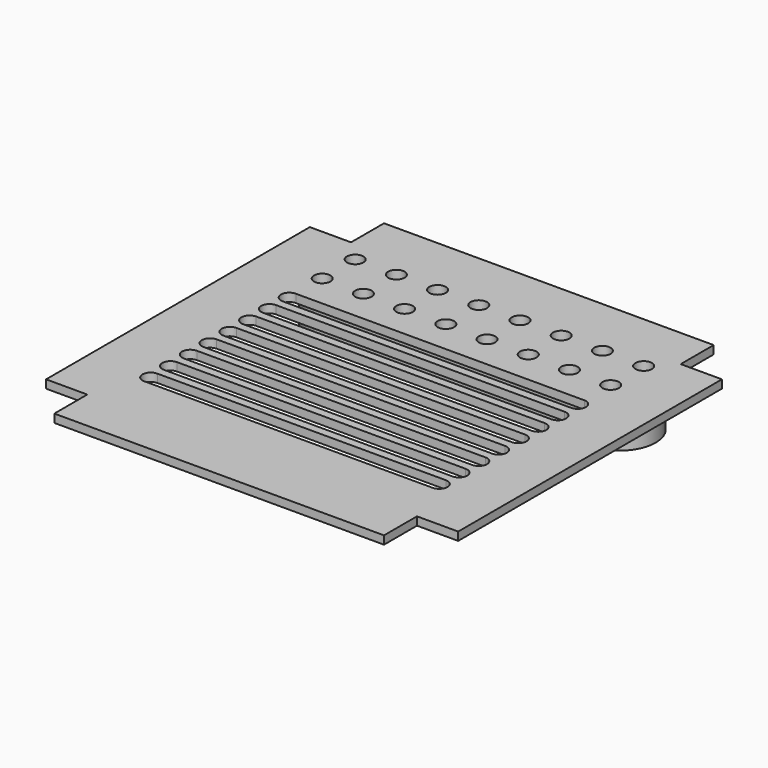
from build123d import *

# Parameters (mm, degrees)
F1_DEPTH = 2.54
F3_DEPTH = 12.7
F4_R     = 2.54
F5_DEPTH = 25.4


# Not quite as in the source:
# - a feature names something its author has since deleted; it is built from what else it names


with BuildPart() as f1:
    # F0 (on Top) → F1 (new body)
    with BuildSketch(Plane.XY):
        Polygon((50.8, 63.5), (0, 63.5), (-50.8, 63.5), (-50.8, 50.8), (-63.5, 50.8), (-63.5, 0), (-63.5, -50.8), (-50.8, -50.8), (-50.8, -63.5), (0, -63.5), (50.8, -63.5), (50.8, -50.8), (63.5, -50.8), (63.5, 0), (63.5, 50.8), (50.8, 50.8), align=None)
    extrude(amount=F1_DEPTH)

    # F2 (on face) → F3 (join)
    with BuildSketch(Plane(origin=(0, 0, 0), x_dir=(1, 0, 0), z_dir=(0, 0, -1))):
        with BuildLine():
            Line((43.2105347984, -26.8235280358), (-43.2105347984, -26.8235280358))
            ThreePointArc((-43.2105347984, -26.8235280358), (-53.3766044151, -38.3837321185), (-42.2611118031, -49.0342304111))
            Line((-42.2611118031, -49.0342304111), (42.2611118031, -49.0342304111))
            ThreePointArc((42.2611118031, -49.0342304111), (53.3766044151, -38.3837321185), (43.2105347984, -26.8235280358))
        make_face()
    extrude(amount=F3_DEPTH)

    # F4 (on face) → F5 (cut)
    with BuildSketch(Plane.XY.offset(2.54)):
        with Locations((-44.45, 44.45)):
            Circle(F4_R)
        with Locations((-44.45, 31.75)):
            Circle(F4_R)
        with Locations((-31.75, 44.45)):
            Circle(F4_R)
        with Locations((-31.75, 31.75)):
            Circle(F4_R)
        with Locations((-19.05, 44.45)):
            Circle(F4_R)
        with Locations((-19.05, 31.75)):
            Circle(F4_R)
        with Locations((-6.35, 44.45)):
            Circle(F4_R)
        with Locations((-6.35, 31.75)):
            Circle(F4_R)
        with Locations((6.35, 44.45)):
            Circle(F4_R)
        with Locations((6.35, 31.75)):
            Circle(F4_R)
        with Locations((19.05, 44.45)):
            Circle(F4_R)
        with Locations((19.05, 31.75)):
            Circle(F4_R)
        with Locations((31.75, 44.45)):
            Circle(F4_R)
        with Locations((31.75, 31.75)):
            Circle(F4_R)
        with Locations((44.45, 44.45)):
            Circle(F4_R)
        with Locations((44.45, 31.75)):
            Circle(F4_R)
        with BuildLine():
            Line((44.45, 21.59), (-44.45, 21.59))
            ThreePointArc((-44.45, 21.59), (-46.99, 19.05), (-44.45, 16.51))
            Line((-44.45, 16.51), (44.45, 16.51))
            ThreePointArc((44.45, 16.51), (46.99, 19.05), (44.45, 21.59))
        make_face()
        with BuildLine():
            Line((44.45, 13.97), (-44.45, 13.97))
            ThreePointArc((-44.45, 13.97), (-46.99, 11.43), (-44.45, 8.89))
            Line((-44.45, 8.89), (44.45, 8.89))
            ThreePointArc((44.45, 8.89), (46.99, 11.43), (44.45, 13.97))
        make_face()
        with BuildLine():
            Line((44.45, 6.35), (-44.45, 6.35))
            ThreePointArc((-44.45, 6.35), (-46.99, 3.81), (-44.45, 1.27))
            Line((-44.45, 1.27), (44.45, 1.27))
            ThreePointArc((44.45, 1.27), (46.99, 3.81), (44.45, 6.35))
        make_face()
        with BuildLine():
            Line((44.45, -1.27), (-44.45, -1.27))
            ThreePointArc((-44.45, -1.27), (-46.99, -3.81), (-44.45, -6.35))
            Line((-44.45, -6.35), (44.45, -6.35))
            ThreePointArc((44.45, -6.35), (46.99, -3.81), (44.45, -1.27))
        make_face()
        with BuildLine():
            Line((44.45, -8.89), (-44.45, -8.89))
            ThreePointArc((-44.45, -8.89), (-46.99, -11.43), (-44.45, -13.97))
            Line((-44.45, -13.97), (44.45, -13.97))
            ThreePointArc((44.45, -13.97), (46.99, -11.43), (44.45, -8.89))
        make_face()
        with BuildLine():
            Line((44.45, -16.51), (-44.45, -16.51))
            ThreePointArc((-44.45, -16.51), (-46.99, -19.05), (-44.45, -21.59))
            Line((-44.45, -21.59), (44.45, -21.59))
            ThreePointArc((44.45, -21.59), (46.99, -19.05), (44.45, -16.51))
        make_face()
        with BuildLine():
            Line((44.45, -24.13), (-44.45, -24.13))
            ThreePointArc((-44.45, -24.13), (-46.99, -26.67), (-44.45, -29.21))
            Line((-44.45, -29.21), (44.45, -29.21))
            ThreePointArc((44.45, -29.21), (46.99, -26.67), (44.45, -24.13))
        make_face()
        with BuildLine():
            Line((44.45, -31.75), (-44.45, -31.75))
            ThreePointArc((-44.45, -31.75), (-46.99, -34.29), (-44.45, -36.83))
            Line((-44.45, -36.83), (44.45, -36.83))
            ThreePointArc((44.45, -36.83), (46.99, -34.29), (44.45, -31.75))
        make_face()
    extrude(amount=-F5_DEPTH, mode=Mode.SUBTRACT)


solid = f1.part
